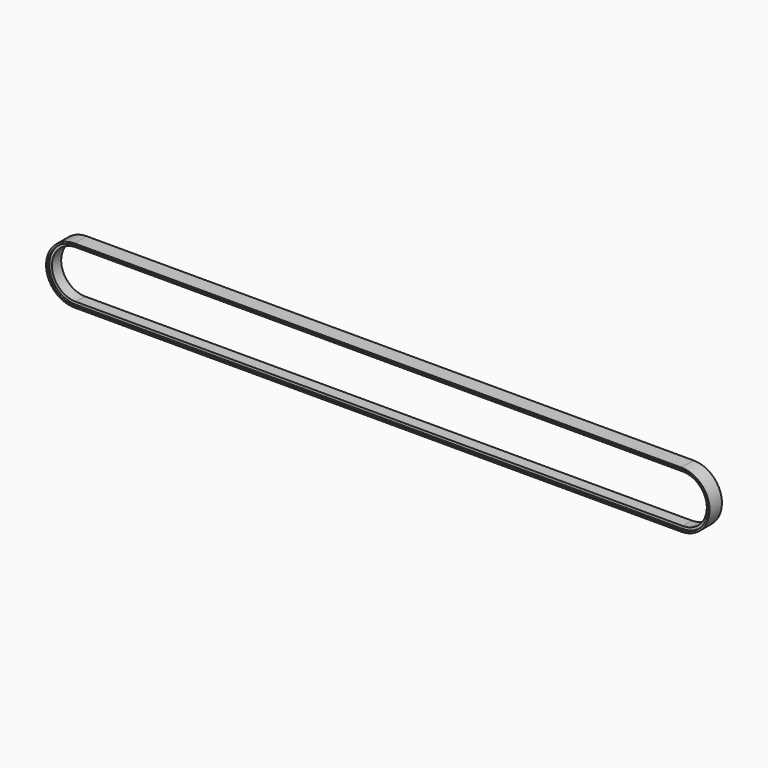
from build123d import *

# Parameters (mm, degrees)
F1_DEPTH = 10
F3_DEPTH = 7.5


with BuildPart() as f1:
    # F0 (on Front) → F1 (new body, symmetric)
    with BuildSketch(Plane.XZ):
        with BuildLine():
            Line((394, 36.7), (-394, 36.7))
            ThreePointArc((-394, 36.7), (-430.7, 0), (-394, -36.7))
            Line((-394, -36.7), (394, -36.7))
            ThreePointArc((394, -36.7), (430.7, 0), (394, 36.7))
        make_face()
        with BuildLine():
            Line((394, -34.5), (-394, -34.5))
            ThreePointArc((-394, -34.5), (-428.5, 0), (-394, 34.5))
            Line((-394, 34.5), (394, 34.5))
            ThreePointArc((394, 34.5), (428.5, 0), (394, -34.5))
        make_face(mode=Mode.SUBTRACT)
    extrude(amount=F1_DEPTH, both=True)

    # F2 (on Front) → F3 (join, symmetric)
    with BuildSketch(Plane.XZ):
        with BuildLine():
            Line((394, 34.5), (-394, 34.5))
            ThreePointArc((-394, 34.5), (-428.5, 0), (-394, -34.5))
            Line((-394, -34.5), (394, -34.5))
            ThreePointArc((394, -34.5), (428.5, 0), (394, 34.5))
        make_face()
        with BuildLine():
            ThreePointArc((-394, -31.1), (-425.1, 0), (-394, 31.1))
            Line((-394, 31.1), (394, 31.1))
            ThreePointArc((394, 31.1), (425.1, 0), (394, -31.1))
            Line((394, -31.1), (-394, -31.1))
        make_face(mode=Mode.SUBTRACT)
    extrude(amount=F3_DEPTH, both=True)


solid = f1.part
